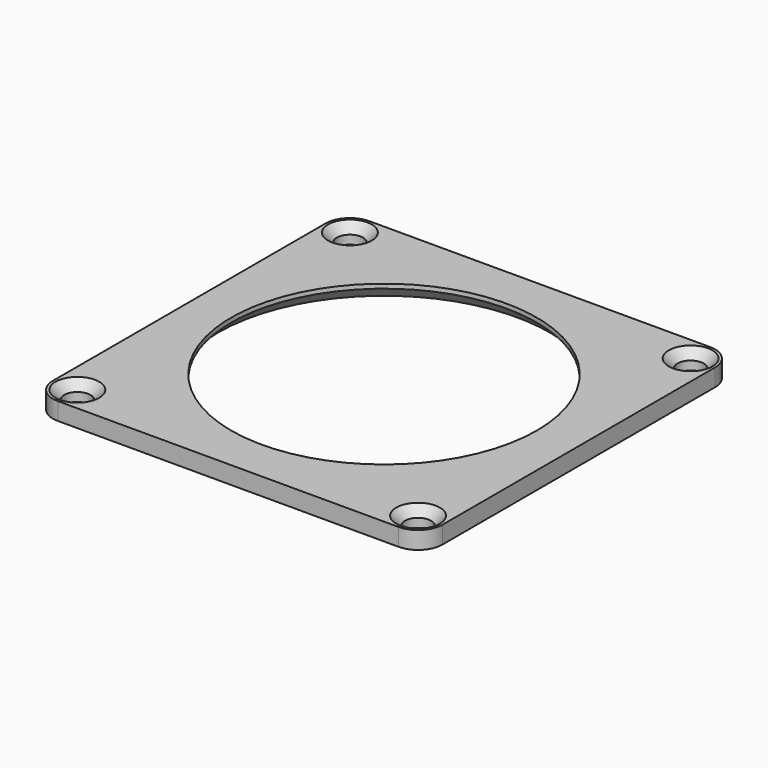
from build123d import *

# Parameters (mm, degrees)
F0_R     = 1.5
F0_R_2   = 19
F0_R_3   = 17.5
F1_DEPTH = 2
F2_SIZE  = 1
F3_SIZE  = 1.5


with BuildPart() as f1:
    # F0 (on Top) → F1 (new body)
    with BuildSketch(Plane.XY):
        with BuildLine():
            Line((-22.3, 19.5), (-22.3, -19.5))
            ThreePointArc((-22.3, -19.5), (-21.4798989873, -21.4798989873), (-19.5, -22.3))
            Line((-19.5, -22.3), (19.5, -22.3))
            ThreePointArc((19.5, -22.3), (21.4798989873, -21.4798989873), (22.3, -19.5))
            Line((22.3, -19.5), (22.3, 19.5))
            ThreePointArc((22.3, 19.5), (21.4798989873, 21.4798989873), (19.5, 22.3))
            Line((19.5, 22.3), (-19.5, 22.3))
            ThreePointArc((-19.5, 22.3), (-21.4798989873, 21.4798989873), (-22.3, 19.5))
        make_face()
        with Locations((-19.5, -19.5)):
            Circle(F0_R, mode=Mode.SUBTRACT)
        with Locations((19.5, -19.5)):
            Circle(F0_R, mode=Mode.SUBTRACT)
        with Locations((-19.5, 19.5)):
            Circle(F0_R, mode=Mode.SUBTRACT)
        Circle(F0_R_2, mode=Mode.SUBTRACT)
        with Locations((19.5, 19.5)):
            Circle(F0_R, mode=Mode.SUBTRACT)
        Circle(F0_R_2)
        Circle(F0_R_3, mode=Mode.SUBTRACT)
    extrude(amount=F1_DEPTH)

    # F2
    f2_edges = [f1.edges().sort_by_distance(p)[0] for p in [
        (-21, 19.5, 2),
        (18, 19.5, 2),
        (18, -19.5, 2),
        (-21, -19.5, 2),
    ]]
    chamfer(f2_edges, length=F2_SIZE)

    # F3
    f3_edges = [f1.edges().sort_by_distance(p)[0] for p in [
        (-17.5, 0, 0),
    ]]
    chamfer(f3_edges, length=F3_SIZE)


solid = f1.part
